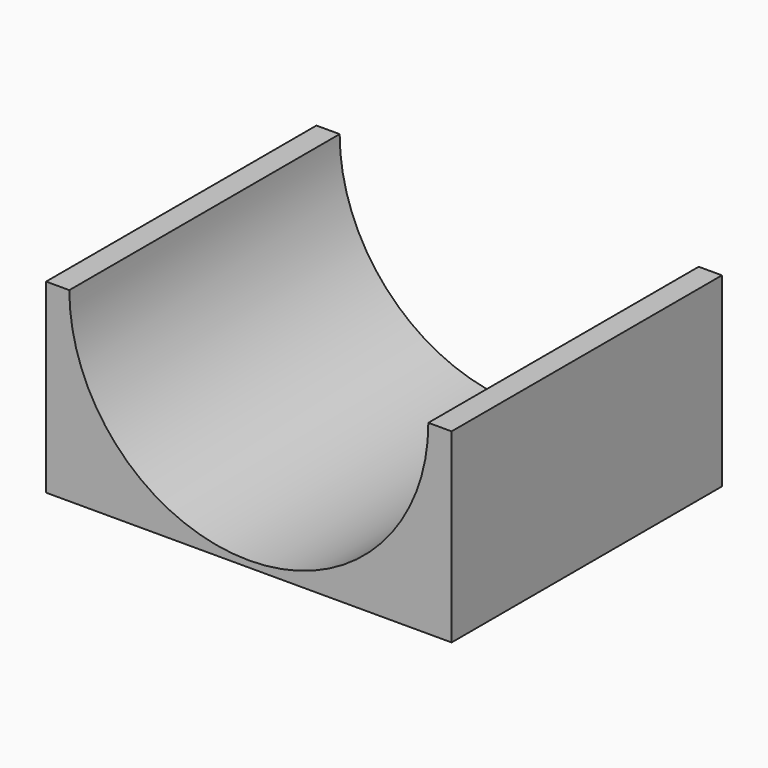
from build123d import *

# Parameters (mm, degrees)
F0_W     = 30.48
F0_H     = 27.94
F1_DEPTH = 12.7
F2_R     = 13.49375
F3_DEPTH = 25.4
F4_W     = 68.546237424
F4_H     = 31.4367190003
F5_DEPTH = 12.7


with BuildPart() as f1:
    # F0 (on Front) → F1 (new body, symmetric)
    with BuildSketch(Plane.XZ):
        Rectangle(F0_W, F0_H)
    extrude(amount=F1_DEPTH, both=True)

    # F2 (on face) → F3 (cut)
    with BuildSketch(Plane.XZ.offset(12.7)):
        Circle(F2_R)
    extrude(amount=-F3_DEPTH, mode=Mode.SUBTRACT)

    # F4 (on Front) → F5 (cut, symmetric)
    with BuildSketch(Plane.XZ):
        with Locations((3.9000464603, 15.7183595002)):
            Rectangle(F4_W, F4_H)
    extrude(amount=F5_DEPTH, both=True, mode=Mode.SUBTRACT)


solid = f1.part
